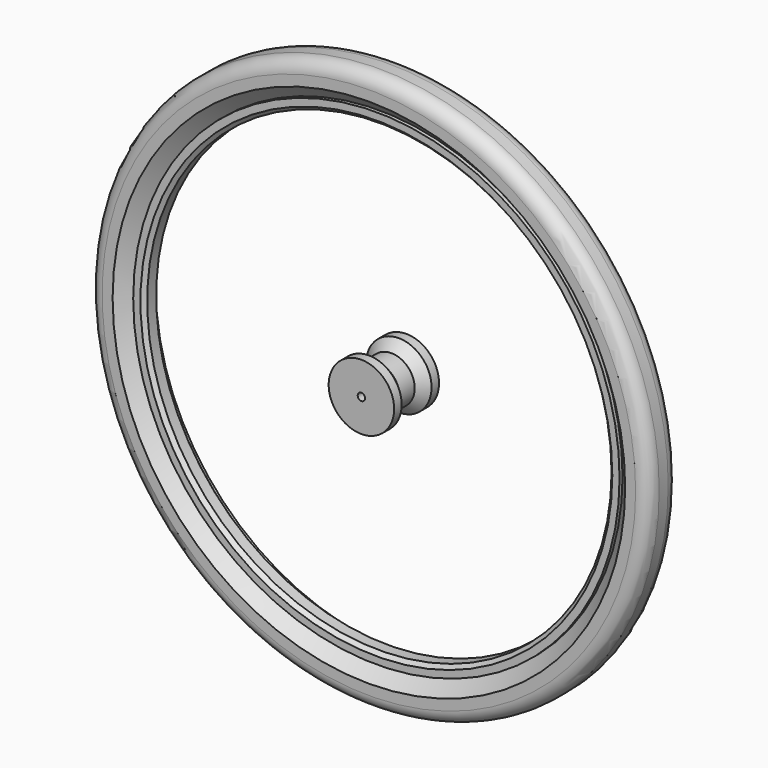
from build123d import *

# Parameters (mm, degrees)
F0_R      = 330.2
F0_R_2    = 315.2659179597
F1_DEPTH  = 12.7
F2_SIZE   = 5.08
F3_R      = 31.75
F4_DEPTH  = 12.7
F5_R      = 44.45
F6_DEPTH  = 25.4
F7_R      = 44.45
F8_DEPTH  = 25.4
F9_SIZE   = 12.69999
F10_R     = 5
F11_DEPTH = 101.6
F12_R     = 379.9884100113
F12_R_2   = 330.2
F13_DEPTH = 25.4
F14_SIZE  = 17.78
F15_R     = 17.78


# Not quite as in the source:
# - a fillet or chamfer is up to 0.001 mm smaller than in the source, because OpenCascade refuses the exact size


with BuildPart() as f1:
    # F0 (on Front) → F1 (new body, symmetric)
    with BuildSketch(Plane.XZ):
        Circle(F0_R)
        Circle(F0_R_2, mode=Mode.SUBTRACT)
    extrude(amount=F1_DEPTH, both=True)

    # F2
    f2_edges = [f1.edges().sort_by_distance(p)[0] for p in [
        (-315.265918, -12.7, 0),
        (-315.265918, 12.7, 0),
    ]]
    chamfer(f2_edges, length=F2_SIZE)


with BuildPart() as f4:
    # F3 (on Front) → F4 (new body, symmetric)
    with BuildSketch(Plane.XZ):
        Circle(F3_R)
    extrude(amount=F4_DEPTH, both=True)

    # F5 (on face) → F6 (join)
    with BuildSketch(Plane.XZ.offset(12.7)):
        Circle(F5_R)
    extrude(amount=F6_DEPTH)

    # F7 (on face) → F8 (join)
    with BuildSketch(Plane(origin=(0, 12.7, 0), x_dir=(-1, 0, 0), z_dir=(0, 1, 0))):
        Circle(F7_R)
    extrude(amount=F8_DEPTH)

    # F9 (size 12.7 in the source; OpenCascade refuses exactly that, so slightly less here)
    f9_edges = [f4.edges().sort_by_distance(p)[0] for p in [
        (-44.45, -12.7, 0),
        (44.45, 12.7, 0),
    ]]
    chamfer(f9_edges, length=F9_SIZE)

    # F10 (on face) → F11 (cut)
    with BuildSketch(Plane.XZ.offset(38.1)):
        Circle(F10_R)
    extrude(amount=-F11_DEPTH, mode=Mode.SUBTRACT)


with BuildPart() as f13:
    # F12 (on Front) → F13 (new body, symmetric)
    with BuildSketch(Plane.XZ):
        Circle(F12_R)
        Circle(F12_R_2, mode=Mode.SUBTRACT)
    extrude(amount=F13_DEPTH, both=True)

    # F14
    f14_edges = [f13.edges().sort_by_distance(p)[0] for p in [
        (-330.2, -25.4, 0),
    ]]
    chamfer(f14_edges, length=F14_SIZE)

    # F15
    f15_edges = [f13.edges().sort_by_distance(p)[0] for p in [
        (-379.98841, -25.4, 0),
        (-379.98841, 25.4, 0),
    ]]
    fillet(f15_edges, radius=F15_R)


solid = Compound([f1.part, f4.part, f13.part])
